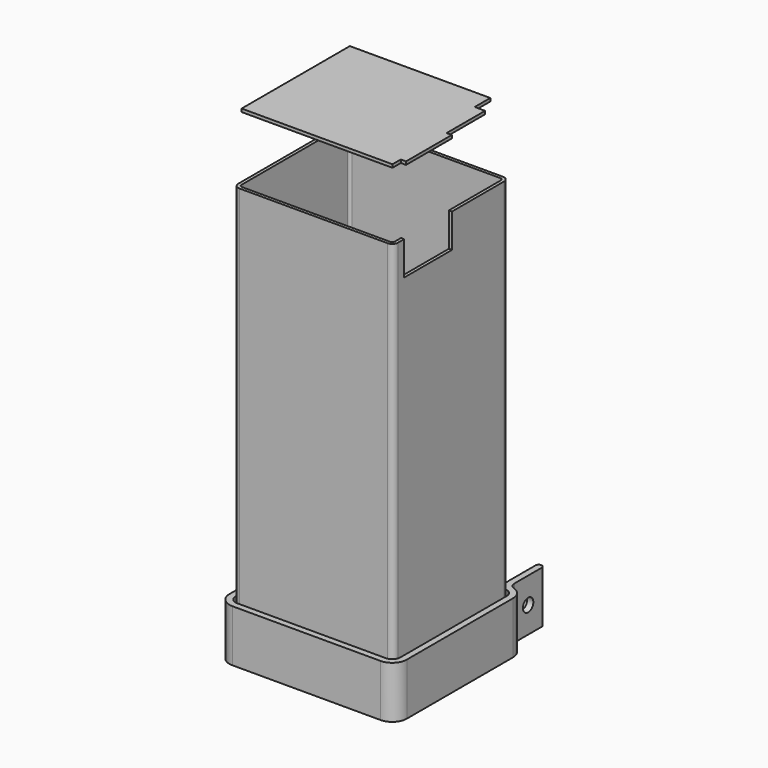
from build123d import *

# Parameters (mm, degrees)
F1_DEPTH      = 160
F1_DEPTH_BACK = 1.2
F2_DEPTH      = 1.2
F3_W          = 23
F3_H          = 13
F4_DEPTH      = 1.2
F6_W          = 0.5
F6_H          = 22
F6_W_2        = 1.5
F7_DEPTH      = 1.2
F8_DEPTH      = 20
F9_R          = 1.19999
F10_R         = 2.5
F11_DEPTH     = 62.501


# Not quite as in the source:
# - a fillet or chamfer is up to 0.001 mm smaller than in the source, because OpenCascade refuses the exact size


with BuildPart() as f1:
    # F0 (on Top) → F1 (new body, two sides)
    with BuildSketch(Plane.XY) as f1_sk:
        with BuildLine():
            Line((-30.7, 25.5), (-30.7, -25.5))
            ThreePointArc((-30.7, -25.5), (-30.0556349186, -27.0556349186), (-28.5, -27.7))
            Line((-28.5, -27.7), (28.5, -27.7))
            ThreePointArc((28.5, -27.7), (30.0556349186, -27.0556349186), (30.7, -25.5))
            Line((30.7, -25.5), (30.7, 25.5))
            ThreePointArc((30.7, 25.5), (30.0556349186, 27.0556349186), (28.5, 27.7))
            Line((28.5, 27.7), (-28.5, 27.7))
            ThreePointArc((-28.5, 27.7), (-30.0556349186, 27.0556349186), (-30.7, 25.5))
        make_face()
        with BuildLine():
            ThreePointArc((29.5, -25.5), (29.2071067812, -26.2071067812), (28.5, -26.5))
            Line((28.5, -26.5), (-28.5, -26.5))
            ThreePointArc((-28.5, -26.5), (-29.2071067812, -26.2071067812), (-29.5, -25.5))
            Line((-29.5, -25.5), (-29.5, 25.5))
            ThreePointArc((-29.5, 25.5), (-29.2071067812, 26.2071067812), (-28.5, 26.5))
            Line((-28.5, 26.5), (28.5, 26.5))
            ThreePointArc((28.5, 26.5), (29.2071067812, 26.2071067812), (29.5, 25.5))
            Line((29.5, 25.5), (29.5, -25.5))
        make_face(mode=Mode.SUBTRACT)
    extrude(amount=F1_DEPTH)
    extrude(f1_sk.sketch, amount=-F1_DEPTH_BACK)

    # F0 (on Top) → F2 (join)
    with BuildSketch(Plane.XY):
        with BuildLine():
            Line((-28.5, -26.5), (28.5, -26.5))
            ThreePointArc((28.5, -26.5), (29.2071067812, -26.2071067812), (29.5, -25.5))
            Line((29.5, -25.5), (29.5, 25.5))
            ThreePointArc((29.5, 25.5), (29.2071067812, 26.2071067812), (28.5, 26.5))
            Line((28.5, 26.5), (-28.5, 26.5))
            ThreePointArc((-28.5, 26.5), (-29.2071067812, 26.2071067812), (-29.5, 25.5))
            Line((-29.5, 25.5), (-29.5, -25.5))
            ThreePointArc((-29.5, -25.5), (-29.2071067812, -26.2071067812), (-28.5, -26.5))
        make_face()
    extrude(amount=-F2_DEPTH)

    # F3 (on face) → F4 (cut, through all)
    with BuildSketch(Plane.YZ.offset(30.7)):
        with Locations((-11, 153.5)):
            Rectangle(F3_W, F3_H)
    extrude(amount=-F4_DEPTH, mode=Mode.SUBTRACT)


with BuildPart() as f7:
    # F6 (on offset) → F7 (new body)
    with BuildSketch(Plane.XY.offset(185)):
        Polygon((29, -22), (29, 0), (29, 18.5), (25, 18.5), (25, 26), (-29, 26), (-29, -26), (29, -26), align=None)
        with Locations((29.25, -11)):
            Rectangle(F6_W, F6_H)
        with Locations((30.25, -11)):
            Rectangle(F6_W_2, F6_H)
    extrude(amount=F7_DEPTH)


with BuildPart() as f8:
    # F0 (on Top) → F8 (new body)
    with BuildSketch(Plane.XY):
        with BuildLine():
            ThreePointArc((29.5024096386, 28.5389430591), (31.0930398033, 27.3751385491), (31.7, 25.5))
            Line((31.7, 25.5), (31.7, -25.5))
            ThreePointArc((31.7, -25.5), (30.7627416998, -27.7627416998), (28.5, -28.7))
            Line((28.5, -28.7), (-28.5, -28.7))
            ThreePointArc((-28.5, -28.7), (-30.7627416998, -27.7627416998), (-31.7, -25.5))
            Line((-31.7, -25.5), (-31.7, 25.5))
            ThreePointArc((-31.7, 25.5), (-31.0930398033, 27.3751385491), (-29.5024096386, 28.5389430591))
            ThreePointArc((-29.5024096386, 28.5389430591), (-26.9673428134, 30.393756497), (-26, 33.3822585596))
            Line((-26, 33.3822585596), (-26, 47.7))
            Line((-26, 47.7), (-28.4, 47.7))
            Line((-28.4, 47.7), (-28.4, 33.3822585596))
            ThreePointArc((-28.4, 33.3822585596), (-28.9121226659, 31.8001104088), (-30.2542168675, 30.8181503534))
            ThreePointArc((-30.2542168675, 30.8181503534), (-33.0378196558, 28.7814924609), (-34.1, 25.5))
            Line((-34.1, 25.5), (-34.1, -25.5))
            ThreePointArc((-34.1, -25.5), (-32.4597979746, -29.4597979746), (-28.5, -31.1))
            Line((-28.5, -31.1), (28.5, -31.1))
            ThreePointArc((28.5, -31.1), (32.4597979746, -29.4597979746), (34.1, -25.5))
            Line((34.1, -25.5), (34.1, 25.5))
            ThreePointArc((34.1, 25.5), (33.0378196558, 28.7814924609), (30.2542168675, 30.8181503534))
            ThreePointArc((30.2542168675, 30.8181503534), (28.9121226659, 31.8001104088), (28.4, 33.3822585596))
            Line((28.4, 33.3822585596), (28.4, 47.7))
            Line((28.4, 47.7), (26, 47.7))
            Line((26, 47.7), (26, 33.3822585596))
            ThreePointArc((26, 33.3822585596), (26.9673428134, 30.393756497), (29.5024096386, 28.5389430591))
        make_face()
    extrude(amount=F8_DEPTH)

    # F9 (radius 1.2 in the source; OpenCascade refuses exactly that, so slightly less here)
    f9_edges = [f8.edges().sort_by_distance(p)[0] for p in [
        (-28.4, 47.7, 10),
        (-26, 47.7, 10),
        (28.4, 47.7, 10),
        (26, 47.7, 10),
    ]]
    fillet(f9_edges, radius=F9_R)

    # F10 (on face) → F11 (cut, through all)
    with BuildSketch(Plane(origin=(-28.4, 0, 0), x_dir=(0, -1, 0), z_dir=(-1, 0, 0))):
        with Locations((-39.9411292798, 10)):
            Circle(F10_R)
    extrude(amount=-F11_DEPTH, mode=Mode.SUBTRACT)


solid = Compound([f1.part, f7.part, f8.part])
